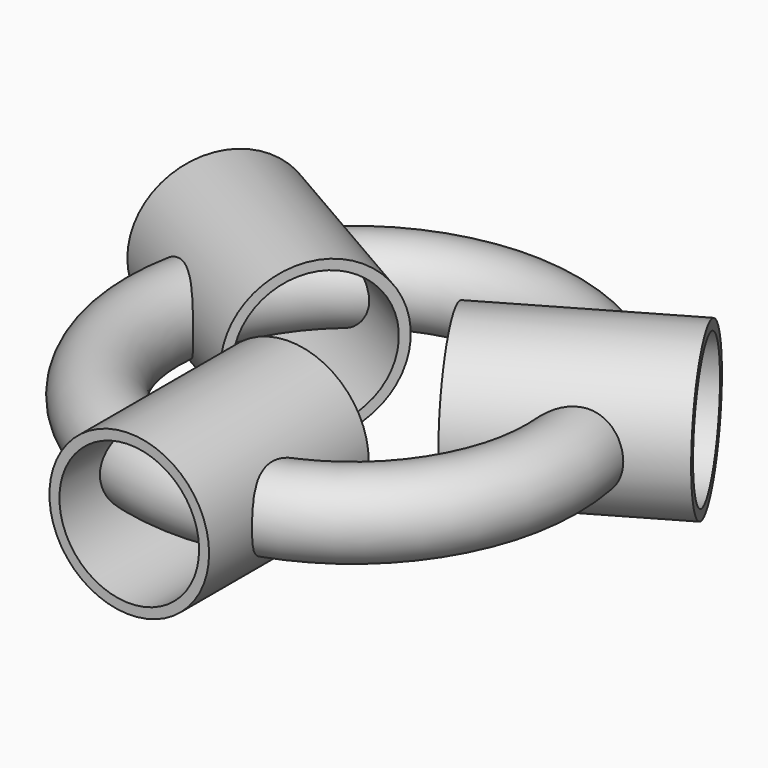
from build123d import *

# Parameters (mm, degrees)
F0_R     = 20
F3_R     = 40
F4_DEPTH = 100
F5_R     = 35
F6_DEPTH = 100
F7_COUNT = 3


with BuildPart() as f1:
    # F0 (on Front) → F1 (revolve)
    with BuildSketch(Plane.XZ):
        with Locations((100, 0)):
            Circle(F0_R)
    revolve(axis=Axis((0, 0, 3.9155493924), (0, 0, -1)))


with BuildPart() as f4:
    # F3 (on offset) → F4 (new body)
    with BuildSketch(Plane.XZ.offset(40)):
        Circle(F3_R)
    extrude(amount=F4_DEPTH)

    # F5 (on face) → F6 (cut)
    with BuildSketch(Plane.XZ.offset(140)):
        Circle(F5_R)
    extrude(amount=-F6_DEPTH, mode=Mode.SUBTRACT)


with BuildPart() as f7_1:
    # F7: instance of F4
    add(f4.part.rotate(Axis((0, 0, 3.9155493924), (0, 0, -1)), 1 * 360 / F7_COUNT))


with BuildPart() as f7_2:
    # F7: instance of F4
    add(f4.part.rotate(Axis((0, 0, 3.9155493924), (0, 0, -1)), 2 * 360 / F7_COUNT))


solid = Compound([f1.part, f4.part, f7_1.part, f7_2.part])
